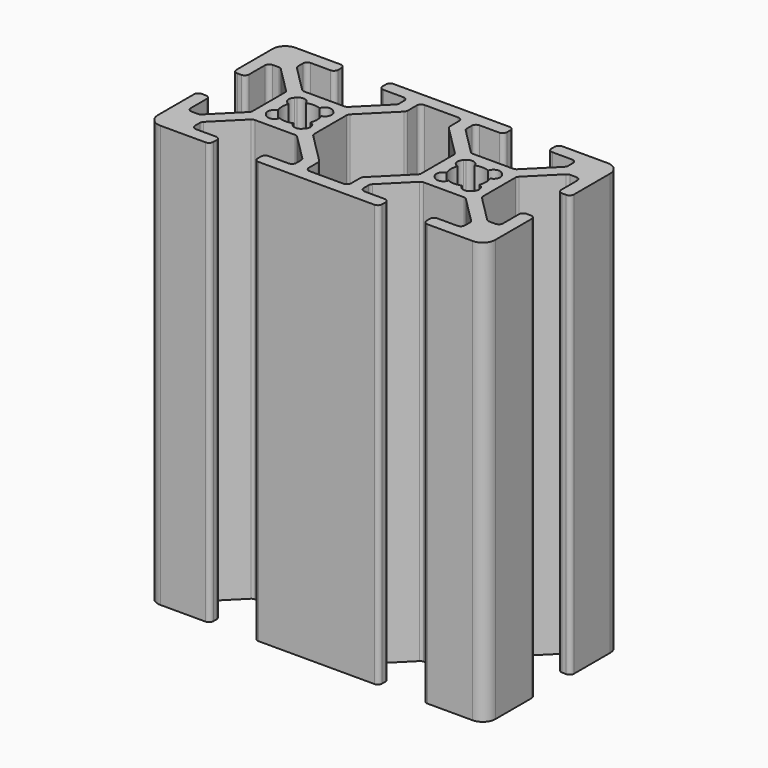
from build123d import *

# Parameters (mm, degrees)
F1_DEPTH = 25


# Not quite as in the source:
# - ends of sketch curves that miss each other by under 0.0002 mm in the source are joined


with BuildPart() as f1:
    # F0 (on Top) → F1 (new body)
    with BuildSketch(Plane.XY):
        with BuildLine():
            ThreePointArc((-6.3715648724, -1.9018951276), (-6.2891612551, -1.8468346664), (-6.1919595, -1.8275))
            Line((-6.1919595, -1.8275), (-3.8080405, -1.8275))
            ThreePointArc((-3.8080405, -1.8275), (-3.7108387449, -1.8468346664), (-3.6284351276, -1.9018951276))
            Line((-3.6284351276, -1.9018951276), (-2.076895, -3.453435))
            ThreePointArc((-2.076895, -3.453435), (-2.0218346664, -3.5358387449), (-2.0025, -3.6330405))
            Line((-2.0025, -3.6330405), (-2.0025, -3.996))
            ThreePointArc((-2.0025, -3.996), (-2.0768948776, -4.1756051224), (-2.2565, -4.25))
            Line((-2.2565, -4.25), (-3.431, -4.25))
            ThreePointArc((-3.431, -4.25), (-3.6106051224, -4.3243948776), (-3.685, -4.504))
            Line((-3.685, -4.504), (-3.685, -4.746))
            ThreePointArc((-3.685, -4.746), (-3.6106051224, -4.9256051224), (-3.431, -5))
            Line((-3.431, -5), (3.431, -5))
            ThreePointArc((3.431, -5), (3.6106051224, -4.9256051224), (3.685, -4.746))
            Line((3.685, -4.746), (3.685, -4.504))
            ThreePointArc((3.685, -4.504), (3.6106051224, -4.3243948776), (3.431, -4.25))
            Line((3.431, -4.25), (2.2565, -4.25))
            ThreePointArc((2.2565, -4.25), (2.0768948776, -4.1756051224), (2.0025, -3.996))
            Line((2.0025, -3.996), (2.0025, -3.6330405))
            ThreePointArc((2.0025, -3.6330405), (2.0218346664, -3.5358387449), (2.0768951276, -3.4534351276))
            Line((2.0768951276, -3.4534351276), (3.628435, -1.901895))
            ThreePointArc((3.628435, -1.901895), (3.7108387449, -1.8468346664), (3.8080405, -1.8275))
            Line((3.8080405, -1.8275), (6.1919595, -1.8275))
            ThreePointArc((6.1919595, -1.8275), (6.2891612551, -1.8468346664), (6.3715648724, -1.9018951276))
            Line((6.3715648724, -1.9018951276), (7.923105, -3.453435))
            ThreePointArc((7.923105, -3.453435), (7.9781653336, -3.5358387449), (7.9975, -3.6330405))
            Line((7.9975, -3.6330405), (7.9975, -3.996))
            ThreePointArc((7.9975, -3.996), (7.9231051224, -4.1756051224), (7.7435, -4.25))
            Line((7.7435, -4.25), (6.569, -4.25))
            ThreePointArc((6.569, -4.25), (6.3893948776, -4.3243948776), (6.315, -4.504))
            Line((6.315, -4.504), (6.315, -4.746))
            ThreePointArc((6.315, -4.746), (6.3893948776, -4.9256051224), (6.569, -5))
            Line((6.569, -5), (9.25, -5))
            ThreePointArc((9.25, -5), (9.7803300859, -4.7803300859), (10, -4.25))
            Line((10, -4.25), (10, -1.569))
            ThreePointArc((10, -1.569), (9.9256051224, -1.3893948776), (9.746, -1.315))
            Line((9.746, -1.315), (9.504, -1.315))
            ThreePointArc((9.504, -1.315), (9.3243948776, -1.3893948776), (9.25, -1.569))
            Line((9.25, -1.569), (9.25, -2.7435))
            ThreePointArc((9.25, -2.7435), (9.1756051224, -2.9231051224), (8.996, -2.9975))
            Line((8.996, -2.9975), (8.6330405, -2.9975))
            ThreePointArc((8.6330405, -2.9975), (8.5358387449, -2.9781653336), (8.4534351276, -2.9231048724))
            Line((8.4534351276, -2.9231048724), (6.901895, -1.371565))
            ThreePointArc((6.901895, -1.371565), (6.8468346664, -1.2891612551), (6.8275, -1.1919595))
            Line((6.8275, -1.1919595), (6.8275, 1.1919595))
            ThreePointArc((6.8275, 1.1919595), (6.8468346664, 1.2891612551), (6.9018951276, 1.3715648724))
            Line((6.9018951276, 1.3715648724), (8.453435, 2.923105))
            ThreePointArc((8.453435, 2.923105), (8.5358387449, 2.9781653336), (8.6330405, 2.9975))
            Line((8.6330405, 2.9975), (8.996, 2.9975))
            ThreePointArc((8.996, 2.9975), (9.1756051224, 2.9231051224), (9.25, 2.7435))
            Line((9.25, 2.7435), (9.25, 1.569))
            ThreePointArc((9.25, 1.569), (9.3243948776, 1.3893948776), (9.504, 1.315))
            Line((9.504, 1.315), (9.746, 1.315))
            ThreePointArc((9.746, 1.315), (9.9256051224, 1.3893948776), (10, 1.569))
            Line((10, 1.569), (10, 4.25))
            ThreePointArc((10, 4.25), (9.7803300859, 4.7803300859), (9.25, 5))
            Line((9.25, 5), (6.569, 5))
            ThreePointArc((6.569, 5), (6.3893948776, 4.9256051224), (6.315, 4.746))
            Line((6.315, 4.746), (6.315, 4.504))
            ThreePointArc((6.315, 4.504), (6.3893948776, 4.3243948776), (6.569, 4.25))
            Line((6.569, 4.25), (7.7435, 4.25))
            ThreePointArc((7.7435, 4.25), (7.9231051224, 4.1756051224), (7.9975, 3.996))
            Line((7.9975, 3.996), (7.9975, 3.6330405))
            ThreePointArc((7.9975, 3.6330405), (7.9781653336, 3.5358387449), (7.9231048724, 3.4534351276))
            Line((7.9231048724, 3.4534351276), (6.371565, 1.901895))
            ThreePointArc((6.371565, 1.901895), (6.2891612551, 1.8468346664), (6.1919595, 1.8275))
            Line((6.1919595, 1.8275), (3.8080405, 1.8275))
            ThreePointArc((3.8080405, 1.8275), (3.7108387449, 1.8468346664), (3.6284351276, 1.9018951276))
            Line((3.6284351276, 1.9018951276), (2.076895, 3.453435))
            ThreePointArc((2.076895, 3.453435), (2.0218346664, 3.5358387449), (2.0025, 3.6330405))
            Line((2.0025, 3.6330405), (2.0025, 3.996))
            ThreePointArc((2.0025, 3.996), (2.0768948776, 4.1756051224), (2.2565, 4.25))
            Line((2.2565, 4.25), (3.431, 4.25))
            ThreePointArc((3.431, 4.25), (3.6106051224, 4.3243948776), (3.685, 4.504))
            Line((3.685, 4.504), (3.685, 4.746))
            ThreePointArc((3.685, 4.746), (3.6106051224, 4.9256051224), (3.431, 5))
            Line((3.431, 5), (-3.431, 5))
            ThreePointArc((-3.431, 5), (-3.6106051224, 4.9256051224), (-3.685, 4.746))
            Line((-3.685, 4.746), (-3.685, 4.504))
            ThreePointArc((-3.685, 4.504), (-3.6106051224, 4.3243948776), (-3.431, 4.25))
            Line((-3.431, 4.25), (-2.2565, 4.25))
            ThreePointArc((-2.2565, 4.25), (-2.0768948776, 4.1756051224), (-2.0025, 3.996))
            Line((-2.0025, 3.996), (-2.0025, 3.6330405))
            ThreePointArc((-2.0025, 3.6330405), (-2.0218346664, 3.5358387449), (-2.0768951276, 3.4534351276))
            Line((-2.0768951276, 3.4534351276), (-3.628435, 1.901895))
            ThreePointArc((-3.628435, 1.901895), (-3.7108387449, 1.8468346664), (-3.8080405, 1.8275))
            Line((-3.8080405, 1.8275), (-6.1919595, 1.8275))
            ThreePointArc((-6.1919595, 1.8275), (-6.2891612551, 1.8468346664), (-6.3715648724, 1.9018951276))
            Line((-6.3715648724, 1.9018951276), (-7.923105, 3.453435))
            ThreePointArc((-7.923105, 3.453435), (-7.9781653336, 3.5358387449), (-7.9975, 3.6330405))
            Line((-7.9975, 3.6330405), (-7.9975, 3.996))
            ThreePointArc((-7.9975, 3.996), (-7.9231051224, 4.1756051224), (-7.7435, 4.25))
            Line((-7.7435, 4.25), (-6.569, 4.25))
            ThreePointArc((-6.569, 4.25), (-6.3893948776, 4.3243948776), (-6.315, 4.504))
            Line((-6.315, 4.504), (-6.315, 4.746))
            ThreePointArc((-6.315, 4.746), (-6.3893948776, 4.9256051224), (-6.569, 5))
            Line((-6.569, 5), (-9.25, 5))
            ThreePointArc((-9.25, 5), (-9.7803300859, 4.7803300859), (-10, 4.25))
            Line((-10, 4.25), (-10, 1.569))
            ThreePointArc((-10, 1.569), (-9.9256051224, 1.3893948776), (-9.746, 1.315))
            Line((-9.746, 1.315), (-9.504, 1.315))
            ThreePointArc((-9.504, 1.315), (-9.3243948776, 1.3893948776), (-9.25, 1.569))
            Line((-9.25, 1.569), (-9.25, 2.7435))
            ThreePointArc((-9.25, 2.7435), (-9.1756051224, 2.9231051224), (-8.996, 2.9975))
            Line((-8.996, 2.9975), (-8.6330405, 2.9975))
            ThreePointArc((-8.6330405, 2.9975), (-8.5358387449, 2.9781653336), (-8.4534351276, 2.9231048724))
            Line((-8.4534351276, 2.9231048724), (-6.901895, 1.371565))
            ThreePointArc((-6.901895, 1.371565), (-6.8468346664, 1.2891612551), (-6.8275, 1.1919595))
            Line((-6.8275, 1.1919595), (-6.8275, -1.1919595))
            ThreePointArc((-6.8275, -1.1919595), (-6.8468346664, -1.2891612551), (-6.9018951276, -1.3715648724))
            Line((-6.9018951276, -1.3715648724), (-8.453435, -2.923105))
            ThreePointArc((-8.453435, -2.923105), (-8.5358387449, -2.9781653336), (-8.6330405, -2.9975))
            Line((-8.6330405, -2.9975), (-8.996, -2.9975))
            ThreePointArc((-8.996, -2.9975), (-9.1756051224, -2.9231051224), (-9.25, -2.7435))
            Line((-9.25, -2.7435), (-9.25, -1.569))
            ThreePointArc((-9.25, -1.569), (-9.3243948776, -1.3893948776), (-9.504, -1.315))
            Line((-9.504, -1.315), (-9.746, -1.315))
            ThreePointArc((-9.746, -1.315), (-9.9256051224, -1.3893948776), (-10, -1.569))
            Line((-10, -1.569), (-10, -4.25))
            ThreePointArc((-10, -4.25), (-9.7803300859, -4.7803300859), (-9.25, -5))
            Line((-9.25, -5), (-6.569, -5))
            ThreePointArc((-6.569, -5), (-6.3893948776, -4.9256051224), (-6.315, -4.746))
            Line((-6.315, -4.746), (-6.315, -4.504))
            ThreePointArc((-6.315, -4.504), (-6.3893948776, -4.3243948776), (-6.569, -4.25))
            Line((-6.569, -4.25), (-7.7435, -4.25))
            ThreePointArc((-7.7435, -4.25), (-7.9231051224, -4.1756051224), (-7.9975, -3.996))
            Line((-7.9975, -3.996), (-7.9975, -3.6330405))
            ThreePointArc((-7.9975, -3.6330405), (-7.9781653336, -3.5358387449), (-7.9231048724, -3.4534351276))
            Line((-7.9231048724, -3.4534351276), (-6.3715648724, -1.9018951276))
        make_face()
        with BuildLine():
            ThreePointArc((-5.4019885069, -0.9675669983), (-5.678234106, -1.2529690728), (-6.0624505184, -1.1522530184))
            Line((-6.0624505184, -1.1522530184), (-6.152253, -1.0624505))
            ThreePointArc((-6.152253, -1.0624505), (-6.2529690728, -0.678234106), (-5.9675669983, -0.4019885069))
            ThreePointArc((-5.9675669983, -0.4019885069), (-6.04775, 0), (-5.9675667395, 0.4019883918))
            ThreePointArc((-5.9675667395, 0.4019883918), (-6.2529690728, 0.678234106), (-6.1522530184, 1.0624505184))
            Line((-6.1522530184, 1.0624505184), (-6.0624505, 1.152253))
            ThreePointArc((-6.0624505, 1.152253), (-5.678234106, 1.2529690728), (-5.4019885069, 0.9675669983))
            ThreePointArc((-5.4019885069, 0.9675669983), (-5, 1.04775), (-4.5980116082, 0.9675667395))
            ThreePointArc((-4.5980116082, 0.9675667395), (-4.321765894, 1.2529690728), (-3.9375494816, 1.1522530184))
            Line((-3.9375494816, 1.1522530184), (-3.847747, 1.0624505))
            ThreePointArc((-3.847747, 1.0624505), (-3.7470309272, 0.678234106), (-4.0324330017, 0.4019885069))
            ThreePointArc((-4.0324330017, 0.4019885069), (-3.95225, 0), (-4.0324332605, -0.4019883918))
            ThreePointArc((-4.0324332605, -0.4019883918), (-3.7470309272, -0.678234106), (-3.8477469816, -1.0624505184))
            Line((-3.8477469816, -1.0624505184), (-3.9375495, -1.152253))
            ThreePointArc((-3.9375495, -1.152253), (-4.321765894, -1.2529690728), (-4.5980114931, -0.9675669983))
            ThreePointArc((-4.5980114931, -0.9675669983), (-5, -1.04775), (-5.4019885069, -0.9675669983))
        make_face(mode=Mode.SUBTRACT)
        with BuildLine():
            ThreePointArc((-0.9985, -4.25), (-1.1781051224, -4.1756051224), (-1.2525, -3.996))
            Line((-1.2525, -3.996), (-1.2525, -3.32238))
            ThreePointArc((-1.2525, -3.32238), (-1.2718345987, -3.2251784082), (-1.3268948776, -3.1427748776))
            Line((-1.3268948776, -3.1427748776), (-3.098105, -1.371565))
            ThreePointArc((-3.098105, -1.371565), (-3.1531653336, -1.2891612551), (-3.1725, -1.1919595))
            Line((-3.1725, -1.1919595), (-3.1725, 1.1919595))
            ThreePointArc((-3.1725, 1.1919595), (-3.1531653336, 1.2891612551), (-3.0981048724, 1.3715648724))
            Line((-3.0981048724, 1.3715648724), (-1.326895, 3.142775))
            ThreePointArc((-1.326895, 3.142775), (-1.2718345987, 3.2251784082), (-1.2525, 3.32238))
            Line((-1.2525, 3.32238), (-1.2525, 3.996))
            ThreePointArc((-1.2525, 3.996), (-1.1781051224, 4.1756051224), (-0.9985, 4.25))
            Line((-0.9985, 4.25), (0.9985, 4.25))
            ThreePointArc((0.9985, 4.25), (1.1781051224, 4.1756051224), (1.2525, 3.996))
            Line((1.2525, 3.996), (1.2525, 3.32238))
            ThreePointArc((1.2525, 3.32238), (1.2718345987, 3.2251784082), (1.3268948776, 3.1427748776))
            Line((1.3268948776, 3.1427748776), (3.098105, 1.371565))
            ThreePointArc((3.098105, 1.371565), (3.1531653336, 1.2891612551), (3.1725, 1.1919595))
            Line((3.1725, 1.1919595), (3.1725, -1.1919595))
            ThreePointArc((3.1725, -1.1919595), (3.1531653336, -1.2891612551), (3.0981048724, -1.3715648724))
            Line((3.0981048724, -1.3715648724), (1.326895, -3.142775))
            ThreePointArc((1.326895, -3.142775), (1.2718345987, -3.2251784082), (1.2525, -3.32238))
            Line((1.2525, -3.32238), (1.2525, -3.996))
            ThreePointArc((1.2525, -3.996), (1.1781051224, -4.1756051224), (0.9985, -4.25))
            Line((0.9985, -4.25), (-0.9985, -4.25))
        make_face(mode=Mode.SUBTRACT)
        with BuildLine():
            ThreePointArc((4.5980114931, -0.9675669983), (4.321765894, -1.2529690728), (3.9375494816, -1.1522530184))
            Line((3.9375494816, -1.1522530184), (3.847747, -1.0624505))
            ThreePointArc((3.847747, -1.0624505), (3.7470309272, -0.678234106), (4.0324330017, -0.4019885069))
            ThreePointArc((4.0324330017, -0.4019885069), (3.95225, 0), (4.0324332605, 0.4019883918))
            ThreePointArc((4.0324332605, 0.4019883918), (3.7470309272, 0.678234106), (3.8477469816, 1.0624505184))
            Line((3.8477469816, 1.0624505184), (3.9375495, 1.152253))
            ThreePointArc((3.9375495, 1.152253), (4.321765894, 1.2529690728), (4.5980114931, 0.9675669983))
            ThreePointArc((4.5980114931, 0.9675669983), (5, 1.04775), (5.4019883918, 0.9675667395))
            ThreePointArc((5.4019883918, 0.9675667395), (5.678234106, 1.2529690728), (6.0624505184, 1.1522530184))
            Line((6.0624505184, 1.1522530184), (6.152253, 1.0624505))
            ThreePointArc((6.152253, 1.0624505), (6.2529690728, 0.678234106), (5.9675669983, 0.4019885069))
            ThreePointArc((5.9675669983, 0.4019885069), (6.04775, 0), (5.9675667395, -0.4019883918))
            ThreePointArc((5.9675667395, -0.4019883918), (6.2529690728, -0.678234106), (6.1522530184, -1.0624505184))
            Line((6.1522530184, -1.0624505184), (6.0624505, -1.152253))
            ThreePointArc((6.0624505, -1.152253), (5.678234106, -1.2529690728), (5.4019885069, -0.9675669983))
            ThreePointArc((5.4019885069, -0.9675669983), (5, -1.04775), (4.5980114931, -0.9675669983))
        make_face(mode=Mode.SUBTRACT)
    extrude(amount=F1_DEPTH)


solid = f1.part
